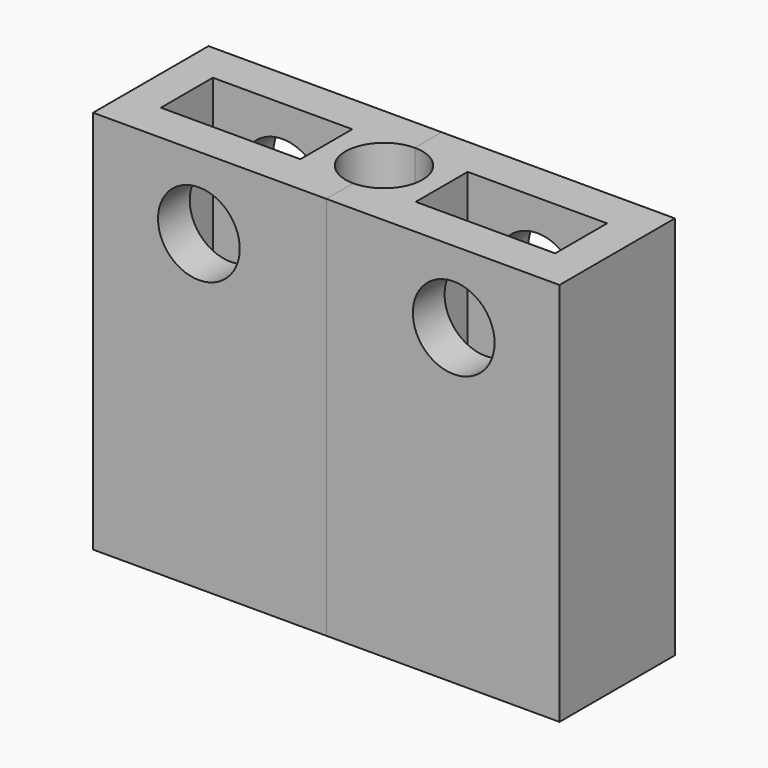
from build123d import *
from build123d import SkipClean  # not in build123d's __all__

# Parameters (mm, degrees)
F1_DEPTH = 16
F2_R     = 1.7
F3_DEPTH = 25


with BuildPart() as f1:
    # F0 (on Top) → F1 (new body)
    with BuildSketch(Plane.XY):
        with BuildLine():
            ThreePointArc((0, -1.6), (-1.6, 0), (0, 1.6))
            Line((0, 1.6), (0, 3))
            Line((0, 3), (-9.7, 3))
            Line((-9.7, 3), (-9.7, 0))
            Line((-9.7, 0), (-9.7, -3))
            Line((-9.7, -3), (0, -3))
            Line((0, -3), (0, -1.6))
        make_face()
        Polygon((-8.2, -1.35), (-8.2, 0), (-8.2, 1.35), (-2.4, 1.35), (-2.4, -1.35), align=None, mode=Mode.SUBTRACT)
    extrude(amount=F1_DEPTH)

    # F2 (on face) → F3 (cut)
    with BuildSketch(Plane(origin=(0, 3, 0), x_dir=(-1, 0, 0), z_dir=(0, 1, 0))):
        with Locations((5.3, 13)):
            Circle(F2_R)
    extrude(amount=-F3_DEPTH, mode=Mode.SUBTRACT)

    # F4: F1 across plane


with BuildPart() as f1_1:
    add(f1.part, clean=False)
    with SkipClean():  # cleaning this boolean's faces spoils the solid; the shape is the same uncleaned
        add(f1.part.mirror(Plane.YZ), clean=False)


solid = f1_1.part
